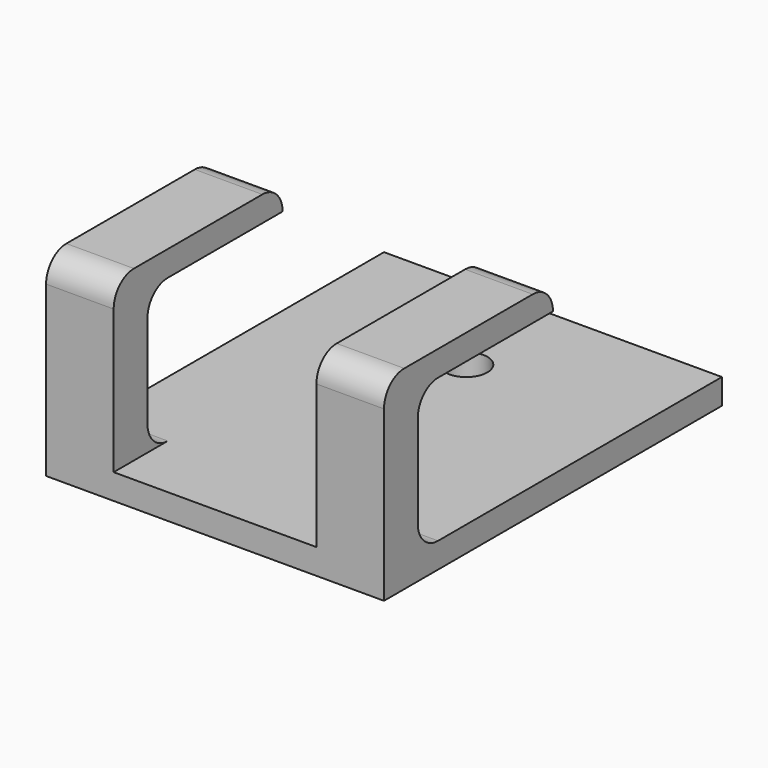
from build123d import *

# Parameters (mm, degrees)
F0_R     = 2.5
F0_W     = 8
F0_H     = 20
F0_H_2   = 5
F0_W_2   = 24
F1_DEPTH = 3
F2_DEPTH = 20
F3_DEPTH = 17
F4_R     = 2.99999


# Not quite as in the source:
# - a fillet or chamfer is up to 0.001 mm smaller than in the source, because OpenCascade refuses the exact size


with BuildPart() as f1:
    # F0 (on Top) → F1 (new body)
    with BuildSketch(Plane.XY):
        Polygon((-5.5937515758, 18.9813033898), (-45.5937515758, 18.9813033898), (-45.5937515758, -6.0186966102), (-37.5937515758, -6.0186966102), (-37.5937515758, -26.0186966102), (-13.5937515758, -26.0186966102), (-13.5937515758, -6.0186966102), (-5.5937515758, -6.0186966102), align=None)
        with Locations((-25.5937515758, -10.5820312165)):
            Circle(F0_R, mode=Mode.SUBTRACT)
        with Locations((-25.5937515758, 6.1523453332)):
            Circle(F0_R, mode=Mode.SUBTRACT)
        with Locations((-41.5937515758, -16.0186966102)):
            Rectangle(F0_W, F0_H)
        with Locations((-41.5937515758, -28.5186966102)):
            Rectangle(F0_W, F0_H_2)
        with Locations((-25.5937515758, -28.5186966102)):
            Rectangle(F0_W_2, F0_H_2)
        with Locations((-9.5937515758, -28.5186966102)):
            Rectangle(F0_W, F0_H_2)
        with Locations((-9.5937515758, -16.0186966102)):
            Rectangle(F0_W, F0_H)
    extrude(amount=-F1_DEPTH)

    # F0 (on Top) → F2 (join)
    with BuildSketch(Plane.XY):
        with Locations((-41.5937515758, -16.0186966102)):
            Rectangle(F0_W, F0_H)
        with Locations((-9.5937515758, -16.0186966102)):
            Rectangle(F0_W, F0_H)
        with Locations((-9.5937515758, -28.5186966102)):
            Rectangle(F0_W, F0_H_2)
        with Locations((-41.5937515758, -28.5186966102)):
            Rectangle(F0_W, F0_H_2)
    extrude(amount=F2_DEPTH)

    # F0 (on Top) → F3 (cut)
    with BuildSketch(Plane.XY):
        with Locations((-41.5937515758, -16.0186966102)):
            Rectangle(F0_W, F0_H)
        with Locations((-9.5937515758, -16.0186966102)):
            Rectangle(F0_W, F0_H)
    extrude(amount=F3_DEPTH, mode=Mode.SUBTRACT)

    # F4 (radius 3 in the source; OpenCascade refuses exactly that, so slightly less here)
    f4_edges = [f1.edges().sort_by_distance(p)[0] for p in [
        (-41.593752, -31.018697, 20),
        (-9.593752, -31.018697, 20),
        (-41.593752, -6.018697, 20),
        (-9.593752, -6.018697, 20),
        (-41.593752, -26.018697, 17),
        (-9.593752, -26.018697, 17),
        (-9.593752, -26.018697, 0),
        (-41.593752, -26.018697, 0),
    ]]
    fillet(f4_edges, radius=F4_R)


solid = f1.part
